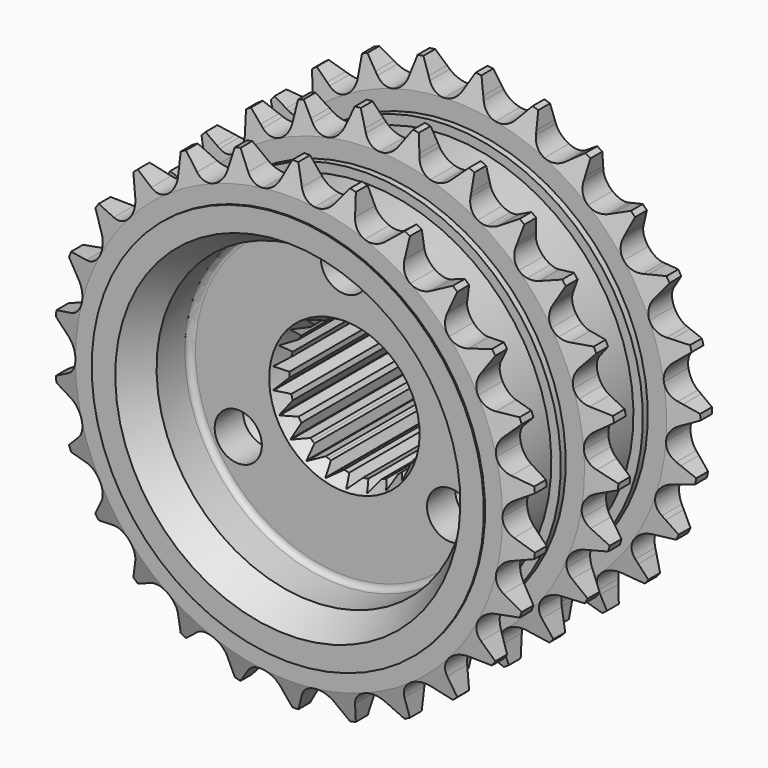
from build123d import *

# Parameters (mm, degrees)
F3_D      = 8
F3_DEPTH  = 6
F3_TIP    = 2.4034424761
F5_DEPTH  = 28.501
F6_R      = 41.9748747762
F7_DEPTH  = 6
F8_R      = 43.059736228
F9_DEPTH  = 6
F10_R     = 43.2062525831
F11_DEPTH = 6


# Not quite as in the source:
# - ends of sketch curves that miss each other by under 0.0002 mm in the source are joined


with BuildPart() as f1:
    # F0 (on Right) → F1 (revolve)
    with BuildSketch(Plane.YZ):
        with BuildLine():
            Line((0, 33.25), (0, 29.25))
            Line((0, 29.25), (5, 26.25))
            Line((5, 26.25), (11, 26.25))
            ThreePointArc((11, 26.25), (11.7071067812, 25.9571067812), (12, 25.25))
            Line((12, 25.25), (12, 12.75))
            Line((12, 12.75), (14.5, 11.35))
            Line((14.5, 11.35), (35.6, 11.35))
            Line((35.6, 11.35), (37, 12.75))
            Line((37, 12.75), (37, 17.5))
            Line((37, 17.5), (34.5, 18.75))
            ThreePointArc((34.5, 18.75), (31.5, 23.25), (34.5, 27.75))
            Line((34.5, 27.75), (37.5, 27.75))
            Line((37.5, 27.75), (40.5, 29.25))
            Line((40.5, 29.25), (40.5, 33.25))
            Line((40.5, 33.25), (40.25, 33.25))
            Line((40.25, 33.25), (40.25, 36.2))
            Line((40.25, 36.2), (38.9, 40.85))
            Line((38.9, 40.85), (36.4, 40.85))
            Line((36.4, 40.85), (35.05, 36.2))
            Line((35.05, 36.2), (35.05, 33))
            Line((35.05, 33), (34, 33))
            Line((34, 33), (34, 31.4))
            Line((34, 31.4), (23.9, 31.4))
            Line((23.9, 31.4), (23.9, 33))
            Line((23.9, 33), (22.85, 33))
            Line((22.85, 33), (22.85, 36.2))
            Line((22.85, 36.2), (21.5, 40.85))
            Line((21.5, 40.85), (19, 40.85))
            Line((19, 40.85), (17.65, 36.2))
            Line((17.65, 36.2), (17.65, 33))
            Line((17.65, 33), (16.6, 33))
            Line((16.6, 33), (16.6, 31.4))
            Line((16.6, 31.4), (6.5, 31.4))
            Line((6.5, 31.4), (6.5, 33))
            Line((6.5, 33), (5.45, 33))
            Line((5.45, 33), (5.45, 36.2))
            Line((5.45, 36.2), (4.1, 40.85))
            Line((4.1, 40.85), (1.6, 40.85))
            Line((1.6, 40.85), (0.25, 36.2))
            Line((0.25, 36.2), (0.25, 33.25))
            Line((0.25, 33.25), (0, 33.25))
        make_face()
    revolve(axis=Axis((0, 20.25, 0), (0, 1, 0)))

    # F3
    with Locations(Plane.XZ.offset(-12)):
        with Locations((0, 20.78), (17.9960078906, -10.39), (-17.9960078906, -10.39)):
            Hole(F3_D / 2, depth=F3_DEPTH)
            with Locations((0, 0, -(F3_DEPTH + F3_TIP / 2))):  # 118° drill point
                Cone(0, F3_D / 2, F3_TIP, mode=Mode.SUBTRACT)

    # F4 (on face) → F5 (cut, through all)
    with BuildSketch(Plane.XZ.offset(-12)):
        with BuildLine():
            Line((1.168584, 11.289682), (0.05, 12.4999))
            ThreePointArc((0.05, 12.4999), (0.02500005, 12.4999749999), (0, 12.5))
            ThreePointArc((0, 12.5), (-0.02500005, 12.4999749999), (-0.05, 12.4998999996))
            Line((-0.05, 12.4998999996), (-1.168584, 11.289682))
            ThreePointArc((-1.168584, 11.289682), (-1.3922022006, 11.2642919455), (-1.6152730599, 11.2344734163))
            ThreePointArc((-1.6152730599, 11.2344734163), (-1.8377093299, 11.2002376947), (-2.0594230559, 11.161598303))
            Line((-2.0594230559, 11.161598303), (-3.473654, 12.007653))
            ThreePointArc((-3.473654, 12.007653), (-3.497662502, 12.0006815232), (-3.5216570429, 11.993662146))
            ThreePointArc((-3.5216570429, 11.993662146), (-3.5456370746, 11.9865949183), (-3.5696029241, 11.9794797452))
            Line((-3.5696029241, 11.9794797452), (-4.301919, 10.503142))
            ThreePointArc((-4.301919, 10.503142), (-4.5093260475, 10.4157802683), (-4.7149601243, 10.3243232721))
            ThreePointArc((-4.7149601243, 10.3243232721), (-4.9187409108, 10.2288067658), (-5.1205877627, 10.1292685306))
            Line((-5.1205877627, 10.1292685306), (-6.715893, 10.542617))
            ThreePointArc((-6.715893, 10.542617), (-6.7369651285, 10.5291643), (-6.7580101367, 10.5156692127))
            ThreePointArc((-6.7580101367, 10.5156692127), (-6.7790281001, 10.5021320701), (-6.800018947, 10.4885529183))
            Line((-6.800018947, 10.4885529183), (-7.086738, 8.865701))
            ThreePointArc((-7.086738, 8.865701), (-7.2611308043, 8.7234442419), (-7.4326689778, 8.5777579744))
            ThreePointArc((-7.4326689778, 8.5777579744), (-7.6012851696, 8.4286988184), (-7.7669127104, 8.2763256914))
            Line((-7.7669127104, 8.2763256914), (-9.414051, 8.223481))
            ThreePointArc((-9.414051, 8.223481), (-9.4304793733, 8.2046364204), (-9.4468699032, 8.1857589161))
            ThreePointArc((-9.4468699032, 8.1857589161), (-9.4632224701, 8.1668488709), (-9.4795371845, 8.1479061585))
            Line((-9.4795371845, 8.1479061585), (-9.297432, 6.510013))
            ThreePointArc((-9.297432, 6.510013), (-9.4246825051, 6.3243861107), (-9.5482278417, 6.1362728983))
            ThreePointArc((-9.5482278417, 6.1362728983), (-9.668018783, 5.9457474561), (-9.7840084989, 5.7528842934))
            Line((-9.7840084989, 5.7528842934), (-11.349538, 5.238128))
            ThreePointArc((-11.349538, 5.238128), (-11.3599916731, 5.2154184096), (-11.3703998244, 5.1926879198))
            ThreePointArc((-11.3703998244, 5.1926879198), (-11.3807624714, 5.1699367084), (-11.3910795953, 5.1471648171))
            Line((-11.3910795953, 5.1471648171), (-10.754903, 3.626922))
            ThreePointArc((-10.754903, 3.626922), (-10.8247020133, 3.4129644481), (-10.8902451009, 3.1976650296))
            ThreePointArc((-10.8902451009, 3.1976650296), (-10.9515066301, 2.9811076013), (-11.0084622745, 2.7633780689))
            Line((-11.0084622745, 2.7633780689), (-12.365553, 1.828412))
            ThreePointArc((-12.365553, 1.828412), (-12.3691854533, 1.803677139), (-12.3727680904, 1.778935013))
            ThreePointArc((-12.3727680904, 1.778935013), (-12.3763012032, 1.7541860017), (-12.379784811, 1.7294299736))
            Line((-12.379784811, 1.7294299736), (-11.341076, 0.45))
            ThreePointArc((-11.341076, 0.45), (-11.3477687274, 0.2250442367), (-11.35, 0))
            ThreePointArc((-11.35, 0), (-11.3477687274, -0.2250442367), (-11.341075787, -0.4499999916))
            Line((-11.341075787, -0.4499999916), (-12.379785, -1.72943))
            ThreePointArc((-12.379785, -1.72943), (-12.3763012032, -1.7541860017), (-12.3727680904, -1.778935013))
            ThreePointArc((-12.3727680904, -1.778935013), (-12.3691854533, -1.803677139), (-12.3655533388, -1.8284120501))
            Line((-12.3655533388, -1.8284120501), (-11.008462, -2.763378))
            ThreePointArc((-11.008462, -2.763378), (-10.9515066301, -2.9811076013), (-10.8902451009, -3.1976650296))
            ThreePointArc((-10.8902451009, -3.1976650296), (-10.8247020133, -3.4129644481), (-10.7549029276, -3.6269219756))
            Line((-10.7549029276, -3.6269219756), (-11.39108, -5.147165))
            ThreePointArc((-11.39108, -5.147165), (-11.3807624714, -5.1699367084), (-11.3703998244, -5.1926879198))
            ThreePointArc((-11.3703998244, -5.1926879198), (-11.3599916731, -5.2154184096), (-11.3495380814, -5.2381280376))
            Line((-11.3495380814, -5.2381280376), (-9.784008, -5.752884))
            ThreePointArc((-9.784008, -5.752884), (-9.668018783, -5.9457474561), (-9.5482278417, -6.1362728983))
            ThreePointArc((-9.5482278417, -6.1362728983), (-9.4246825051, -6.3243861107), (-9.2974316011, -6.5100127207))
            Line((-9.2974316011, -6.5100127207), (-9.479537, -8.147906))
            ThreePointArc((-9.479537, -8.147906), (-9.4632224701, -8.1668488709), (-9.4468699032, -8.1857589161))
            ThreePointArc((-9.4468699032, -8.1857589161), (-9.4304793733, -8.2046364204), (-9.4140511209, -8.2234811056))
            Line((-9.4140511209, -8.2234811056), (-7.766913, -8.276326))
            ThreePointArc((-7.766913, -8.276326), (-7.6012851696, -8.4286988184), (-7.4326689778, -8.5777579744))
            ThreePointArc((-7.4326689778, -8.5777579744), (-7.2611308043, -8.7234442419), (-7.0867377331, -8.8657006661))
            Line((-7.0867377331, -8.8657006661), (-6.800019, -10.488553))
            ThreePointArc((-6.800019, -10.488553), (-6.7790281001, -10.5021320701), (-6.7580101367, -10.5156692127))
            ThreePointArc((-6.7580101367, -10.5156692127), (-6.7369651285, -10.5291643), (-6.715893172, -10.54261727))
            Line((-6.715893172, -10.54261727), (-5.120588, -10.129269))
            ThreePointArc((-5.120588, -10.129269), (-4.9187409108, -10.2288067658), (-4.7149601243, -10.3243232721))
            ThreePointArc((-4.7149601243, -10.3243232721), (-4.5093260475, -10.4157802683), (-4.3019190175, -10.5031420426))
            Line((-4.3019190175, -10.5031420426), (-3.569603, -11.97948))
            ThreePointArc((-3.569603, -11.97948), (-3.5456370746, -11.9865949183), (-3.5216570429, -11.993662146))
            ThreePointArc((-3.5216570429, -11.993662146), (-3.497662502, -12.0006815232), (-3.4736539702, -12.007652897))
            Line((-3.4736539702, -12.007652897), (-2.059423, -11.161598))
            ThreePointArc((-2.059423, -11.161598), (-1.8377093299, -11.2002376947), (-1.6152730599, -11.2344734163))
            ThreePointArc((-1.6152730599, -11.2344734163), (-1.3922022006, -11.2642919455), (-1.1685839627, -11.2896816395))
            Line((-1.1685839627, -11.2896816395), (-0.05, -12.4999))
            ThreePointArc((-0.05, -12.4999), (-0.02500005, -12.4999749999), (0, -12.5))
            ThreePointArc((0, -12.5), (0.02500005, -12.4999749999), (0.05, -12.4998999996))
            Line((0.05, -12.4998999996), (1.168584, -11.289682))
            ThreePointArc((1.168584, -11.289682), (1.3922022006, -11.2642919455), (1.6152730599, -11.2344734163))
            ThreePointArc((1.6152730599, -11.2344734163), (1.8377093299, -11.2002376947), (2.0594230559, -11.161598303))
            Line((2.0594230559, -11.161598303), (3.473654, -12.007653))
            ThreePointArc((3.473654, -12.007653), (3.497662502, -12.0006815232), (3.5216570429, -11.993662146))
            ThreePointArc((3.5216570429, -11.993662146), (3.5456370746, -11.9865949183), (3.5696029241, -11.9794797452))
            Line((3.5696029241, -11.9794797452), (4.301919, -10.503142))
            ThreePointArc((4.301919, -10.503142), (4.5093260475, -10.4157802683), (4.7149601243, -10.3243232721))
            ThreePointArc((4.7149601243, -10.3243232721), (4.9187409108, -10.2288067658), (5.1205877627, -10.1292685306))
            Line((5.1205877627, -10.1292685306), (6.715893, -10.542617))
            ThreePointArc((6.715893, -10.542617), (6.7369651285, -10.5291643), (6.7580101367, -10.5156692127))
            ThreePointArc((6.7580101367, -10.5156692127), (6.7790281001, -10.5021320701), (6.800018947, -10.4885529183))
            Line((6.800018947, -10.4885529183), (7.086738, -8.865701))
            ThreePointArc((7.086738, -8.865701), (7.2611308043, -8.7234442419), (7.4326689778, -8.5777579744))
            ThreePointArc((7.4326689778, -8.5777579744), (7.6012851696, -8.4286988184), (7.7669127104, -8.2763256914))
            Line((7.7669127104, -8.2763256914), (9.414051, -8.223481))
            ThreePointArc((9.414051, -8.223481), (9.4304793733, -8.2046364204), (9.4468699032, -8.1857589161))
            ThreePointArc((9.4468699032, -8.1857589161), (9.4632224701, -8.1668488709), (9.4795371845, -8.1479061585))
            Line((9.4795371845, -8.1479061585), (9.297432, -6.510013))
            ThreePointArc((9.297432, -6.510013), (9.4246825051, -6.3243861107), (9.5482278417, -6.1362728983))
            ThreePointArc((9.5482278417, -6.1362728983), (9.668018783, -5.9457474561), (9.7840084989, -5.7528842934))
            Line((9.7840084989, -5.7528842934), (11.349538, -5.238128))
            ThreePointArc((11.349538, -5.238128), (11.3599916731, -5.2154184096), (11.3703998244, -5.1926879198))
            ThreePointArc((11.3703998244, -5.1926879198), (11.3807624714, -5.1699367084), (11.3910795953, -5.1471648171))
            Line((11.3910795953, -5.1471648171), (10.754903, -3.626922))
            ThreePointArc((10.754903, -3.626922), (10.8247020133, -3.4129644481), (10.8902451009, -3.1976650296))
            ThreePointArc((10.8902451009, -3.1976650296), (10.9515066301, -2.9811076013), (11.0084622745, -2.7633780689))
            Line((11.0084622745, -2.7633780689), (12.365553, -1.828412))
            ThreePointArc((12.365553, -1.828412), (12.3691854533, -1.803677139), (12.3727680904, -1.778935013))
            ThreePointArc((12.3727680904, -1.778935013), (12.3763012032, -1.7541860017), (12.379784811, -1.7294299736))
            Line((12.379784811, -1.7294299736), (11.341076, -0.45))
            ThreePointArc((11.341076, -0.45), (11.3477687274, -0.2250442367), (11.35, 0))
            ThreePointArc((11.35, 0), (11.3477687274, 0.2250442367), (11.341075787, 0.4499999916))
            Line((11.341075787, 0.4499999916), (12.379785, 1.72943))
            ThreePointArc((12.379785, 1.72943), (12.3763012032, 1.7541860017), (12.3727680904, 1.778935013))
            ThreePointArc((12.3727680904, 1.778935013), (12.3691854533, 1.803677139), (12.3655533388, 1.8284120501))
            Line((12.3655533388, 1.8284120501), (11.008462, 2.763378))
            ThreePointArc((11.008462, 2.763378), (10.9515066301, 2.9811076013), (10.8902451009, 3.1976650296))
            ThreePointArc((10.8902451009, 3.1976650296), (10.8247020133, 3.4129644481), (10.7549029276, 3.6269219756))
            Line((10.7549029276, 3.6269219756), (11.39108, 5.147165))
            ThreePointArc((11.39108, 5.147165), (11.3807624714, 5.1699367084), (11.3703998244, 5.1926879198))
            ThreePointArc((11.3703998244, 5.1926879198), (11.3599916731, 5.2154184096), (11.3495380814, 5.2381280376))
            Line((11.3495380814, 5.2381280376), (9.784008, 5.752884))
            ThreePointArc((9.784008, 5.752884), (9.668018783, 5.9457474561), (9.5482278417, 6.1362728983))
            ThreePointArc((9.5482278417, 6.1362728983), (9.4246825051, 6.3243861107), (9.2974316011, 6.5100127207))
            Line((9.2974316011, 6.5100127207), (9.479537, 8.147906))
            ThreePointArc((9.479537, 8.147906), (9.4632224701, 8.1668488709), (9.4468699032, 8.1857589161))
            ThreePointArc((9.4468699032, 8.1857589161), (9.4304793733, 8.2046364204), (9.4140511209, 8.2234811056))
            Line((9.4140511209, 8.2234811056), (7.766913, 8.276326))
            ThreePointArc((7.766913, 8.276326), (7.6012851696, 8.4286988184), (7.4326689778, 8.5777579744))
            ThreePointArc((7.4326689778, 8.5777579744), (7.2611308043, 8.7234442419), (7.0867377331, 8.8657006661))
            Line((7.0867377331, 8.8657006661), (6.800019, 10.488553))
            ThreePointArc((6.800019, 10.488553), (6.7790281001, 10.5021320701), (6.7580101367, 10.5156692127))
            ThreePointArc((6.7580101367, 10.5156692127), (6.7369651285, 10.5291643), (6.715893172, 10.54261727))
            Line((6.715893172, 10.54261727), (5.120588, 10.129269))
            ThreePointArc((5.120588, 10.129269), (4.9187409108, 10.2288067658), (4.7149601243, 10.3243232721))
            ThreePointArc((4.7149601243, 10.3243232721), (4.5093260475, 10.4157802683), (4.3019190175, 10.5031420426))
            Line((4.3019190175, 10.5031420426), (3.569603, 11.97948))
            ThreePointArc((3.569603, 11.97948), (3.5456370746, 11.9865949183), (3.5216570429, 11.993662146))
            ThreePointArc((3.5216570429, 11.993662146), (3.497662502, 12.0006815232), (3.4736539702, 12.007652897))
            Line((3.4736539702, 12.007652897), (2.059423, 11.161598))
            ThreePointArc((2.059423, 11.161598), (1.8377093299, 11.2002376947), (1.6152730599, 11.2344734163))
            ThreePointArc((1.6152730599, 11.2344734163), (1.3922022006, 11.2642919455), (1.168584, 11.289682))
        make_face()
    extrude(amount=-F5_DEPTH, mode=Mode.SUBTRACT)

    # F6 (on face) → F7 (cut)
    with BuildSketch(Plane.XZ.offset(-0.25)):
        Circle(F6_R)
        with BuildLine():
            ThreePointArc((0, 40.85), (0.2500046815, 40.8492349703), (0.4999999989, 40.8469399099))
            Line((0.4999999989, 40.8469399099), (1.816578, 37.832086))
            ThreePointArc((1.816578, 37.832086), (2.8382605046, 36.5459186619), (4.3634280667, 35.936061549))
            ThreePointArc((4.3634280667, 35.936061549), (5.9902249889, 36.1632008832), (7.290019463, 37.1674897438))
            Line((7.290019463, 37.1674897438), (9.2898416715, 39.779659992))
            ThreePointArc((9.2898416715, 39.779659992), (9.5331218028, 39.722060479), (9.7760448861, 39.6629732419))
            ThreePointArc((9.7760448861, 39.6629732419), (10.0186018024, 39.6024004061), (10.2607834663, 39.5403442405))
            Line((10.2607834663, 39.5403442405), (10.8176023373, 36.2980187671))
            ThreePointArc((10.8176023373, 36.2980187671), (11.5017966143, 34.804720487), (12.8366972187, 33.8475882252))
            ThreePointArc((12.8366972187, 33.8475882252), (14.4705803796, 33.678809317), (15.9729472444, 34.3428541905))
            Line((15.9729472444, 34.3428541905), (18.5397915123, 36.4005307385))
            ThreePointArc((18.5397915123, 36.4005307385), (18.7622178993, 36.2863842164), (18.983941578, 36.1708786479))
            ThreePointArc((18.983941578, 36.1708786479), (19.2049542026, 36.0540182792), (19.425247495, 35.9358074872))
            Line((19.425247495, 35.9358074872), (19.1899469471, 32.6544426213))
            ThreePointArc((19.1899469471, 32.6544426213), (19.496890112, 31.0407984674), (20.563944188, 29.7920161047))
            ThreePointArc((20.563944188, 29.7920161047), (22.1099582371, 29.2371277708), (23.7275853913, 29.5223367829))
            Line((23.7275853913, 29.5223367829), (26.7122760597, 30.905934949))
            ThreePointArc((26.7122760597, 30.905934949), (26.9009220894, 30.7418751988), (27.0885605891, 30.5766640628))
            ThreePointArc((27.0885605891, 30.5766640628), (27.2751844718, 30.4103076609), (27.4607867473, 30.2428122241))
            Line((27.4607867473, 30.2428122241), (26.447041593, 27.1131089645))
            ThreePointArc((26.447041593, 27.1131089645), (26.3588952248, 25.4728980696), (27.0960894679, 24.0050402978))
            ThreePointArc((27.0960894679, 24.0050402978), (28.4643856883, 23.0962906312), (30.1032625215, 22.9860884708))
            Line((30.1032625215, 22.9860884708), (33.3323402178, 23.6151985588))
            ThreePointArc((33.3323402178, 23.6151985588), (33.4762424686, 23.4107601368), (33.6188909218, 23.205444904))
            ThreePointArc((33.6188909218, 23.205444904), (33.7602801607, 22.9992604983), (33.9004048897, 22.7922146426))
            Line((33.9004048897, 22.7922146426), (32.1671303126, 19.9960599668))
            ThreePointArc((32.1671303126, 19.9960599668), (31.6890171577, 18.4246054262), (32.0535085182, 16.8229788035))
            ThreePointArc((32.0535085182, 16.8229788035), (33.1645665071, 15.6131810318), (34.7294474548, 15.1139722478))
            Line((34.7294474548, 15.1139722478), (38.0152499205, 14.9520326661))
            ThreePointArc((38.0152499205, 14.9520326661), (38.1060453167, 14.7190967904), (38.1954135137, 14.4856096357))
            ThreePointArc((38.1954135137, 14.4856096357), (38.2833510803, 14.2515799145), (38.3698547229, 14.0170163925))
            Line((38.3698547229, 14.0170163925), (36.0177823412, 11.7169126465))
            ThreePointArc((36.0177823412, 11.7169126465), (35.1774885984, 10.3055416862), (35.1480941632, 8.6632269302))
            ThreePointArc((35.1480941632, 8.6632269302), (35.9373432688, 7.2226901023), (37.3372831385, 6.3634868948))
            Line((37.3372831385, 6.3634868948), (40.4888514776, 5.4199089832))
            ThreePointArc((40.4888514776, 5.4199089832), (40.5212633208, 5.1720130402), (40.5521575069, 4.9239233884))
            ThreePointArc((40.5521575069, 4.9239233884), (40.5815327895, 4.6756493084), (40.6093880683, 4.4272000994))
            Line((40.6093880683, 4.4272000994), (37.7752117794, 2.7568209525))
            ThreePointArc((37.7752117794, 2.7568209525), (36.6215722667, 1.5875573225), (36.2000003336, -2.027e-07))
            ThreePointArc((36.2000003336, -2.027e-07), (36.6215722667, -1.5875573225), (37.7752116417, -2.7568211861))
            Line((37.7752116417, -2.7568211861), (40.6093881579, -4.4272001091))
            ThreePointArc((40.6093881579, -4.4272001091), (40.5815327895, -4.6756493084), (40.5521575069, -4.9239233884))
            ThreePointArc((40.5521575069, -4.9239233884), (40.5212633208, -5.1720130402), (40.4888513883, -5.4199089713))
            Line((40.4888513883, -5.4199089713), (37.3372832163, -6.3634871547))
            ThreePointArc((37.3372832163, -6.3634871547), (35.9373432688, -7.2226901023), (35.1480940662, -8.6632273238))
            ThreePointArc((35.1480940662, -8.6632273238), (35.1774885984, -10.3055416862), (36.0177821515, -11.7169128404))
            Line((36.0177821515, -11.7169128404), (38.3698548075, -14.0170164234))
            ThreePointArc((38.3698548075, -14.0170164234), (38.2833510803, -14.2515799145), (38.1954135137, -14.4856096357))
            ThreePointArc((38.1954135137, -14.4856096357), (38.1060453167, -14.7190967904), (38.0152498366, -14.9520326331))
            Line((38.0152498366, -14.9520326331), (34.7294474682, -15.1139725187))
            ThreePointArc((34.7294474682, -15.1139725187), (33.1645665071, -15.6131810318), (32.0535083298, -16.8229791625))
            ThreePointArc((32.0535083298, -16.8229791625), (31.6890171577, -18.4246054262), (32.1671300821, -19.9960601097))
            Line((32.1671300821, -19.9960601097), (33.9004049645, -22.7922146929))
            ThreePointArc((33.9004049645, -22.7922146929), (33.7602801607, -22.9992604983), (33.6188909218, -23.205444904))
            ThreePointArc((33.6188909218, -23.205444904), (33.4762424686, -23.4107601368), (33.3323401442, -23.6151985067))
            Line((33.3323401442, -23.6151985067), (30.1032624696, -22.986088737))
            ThreePointArc((30.1032624696, -22.986088737), (28.4643856883, -23.0962906312), (27.096089199, -24.0050406012))
            ThreePointArc((27.096089199, -24.0050406012), (26.3588952248, -25.4728980696), (26.447041335, -27.113109048))
            Line((26.447041335, -27.113109048), (27.4607868079, -30.2428122908))
            ThreePointArc((27.4607868079, -30.2428122908), (27.2751844718, -30.4103076609), (27.0885605891, -30.5766640628))
            ThreePointArc((27.0885605891, -30.5766640628), (26.9009220894, -30.7418751988), (26.7122760008, -30.9059348808))
            Line((26.7122760008, -30.9059348808), (23.7275852772, -29.522337029))
            ThreePointArc((23.7275852772, -29.522337029), (22.1099582371, -29.2371277708), (20.5639438543, -29.792016335))
            ThreePointArc((20.5639438543, -29.792016335), (19.496890112, -31.0407984674), (19.1899466766, -32.6544426407))
            Line((19.1899466766, -32.6544426407), (19.4252475379, -35.9358075665))
            ThreePointArc((19.4252475379, -35.9358075665), (19.2049542026, -36.0540182792), (18.983941578, -36.1708786479))
            ThreePointArc((18.983941578, -36.1708786479), (18.7622178993, -36.2863842164), (18.5397914713, -36.4005306582))
            Line((18.5397914713, -36.4005306582), (15.9729470748, -34.3428544022))
            ThreePointArc((15.9729470748, -34.3428544022), (14.4705803796, -33.678809317), (12.8366968397, -33.847588369))
            ThreePointArc((12.8366968397, -33.847588369), (11.5017966143, -34.804720487), (10.81760207, -36.2980187212))
            Line((10.81760207, -36.2980187212), (10.2607834889, -39.5403443277))
            ThreePointArc((10.2607834889, -39.5403443277), (10.0186018024, -39.6024004061), (9.7760448861, -39.6629732419))
            ThreePointArc((9.7760448861, -39.6629732419), (9.5331218028, -39.722060479), (9.289841651, -39.7796599043))
            Line((9.289841651, -39.7796599043), (7.2900192477, -37.1674899087))
            ThreePointArc((7.2900192477, -37.1674899087), (5.9902249889, -36.1632008832), (4.3634276642, -35.9360615979))
            ThreePointArc((4.3634276642, -35.9360615979), (2.8382605046, -36.5459186619), (1.8165777515, -37.8320858915))
            Line((1.8165777515, -37.8320858915), (0.5, -40.84694))
            ThreePointArc((0.5, -40.84694), (0.2500046815, -40.8492349703), (0, -40.85))
            ThreePointArc((0, -40.85), (-0.2500046815, -40.8492349703), (-0.4999999989, -40.8469399099))
            Line((-0.4999999989, -40.8469399099), (-1.816578, -37.832086))
            ThreePointArc((-1.816578, -37.832086), (-2.8382605046, -36.5459186619), (-4.3634280667, -35.936061549))
            ThreePointArc((-4.3634280667, -35.936061549), (-5.9902249889, -36.1632008832), (-7.290019463, -37.1674897438))
            Line((-7.290019463, -37.1674897438), (-9.2898416715, -39.779659992))
            ThreePointArc((-9.2898416715, -39.779659992), (-9.5331218028, -39.722060479), (-9.7760448861, -39.6629732419))
            ThreePointArc((-9.7760448861, -39.6629732419), (-10.0186018024, -39.6024004061), (-10.2607834663, -39.5403442405))
            Line((-10.2607834663, -39.5403442405), (-10.8176023373, -36.2980187671))
            ThreePointArc((-10.8176023373, -36.2980187671), (-11.5017966143, -34.804720487), (-12.8366972187, -33.8475882252))
            ThreePointArc((-12.8366972187, -33.8475882252), (-14.4705803796, -33.678809317), (-15.9729472444, -34.3428541905))
            Line((-15.9729472444, -34.3428541905), (-18.5397915123, -36.4005307385))
            ThreePointArc((-18.5397915123, -36.4005307385), (-18.7622178993, -36.2863842164), (-18.983941578, -36.1708786479))
            ThreePointArc((-18.983941578, -36.1708786479), (-19.2049542026, -36.0540182792), (-19.425247495, -35.9358074872))
            Line((-19.425247495, -35.9358074872), (-19.1899469471, -32.6544426213))
            ThreePointArc((-19.1899469471, -32.6544426213), (-19.496890112, -31.0407984674), (-20.563944188, -29.7920161047))
            ThreePointArc((-20.563944188, -29.7920161047), (-22.1099582371, -29.2371277708), (-23.7275853913, -29.5223367829))
            Line((-23.7275853913, -29.5223367829), (-26.7122760597, -30.905934949))
            ThreePointArc((-26.7122760597, -30.905934949), (-26.9009220894, -30.7418751988), (-27.0885605891, -30.5766640628))
            ThreePointArc((-27.0885605891, -30.5766640628), (-27.2751844718, -30.4103076609), (-27.4607867473, -30.2428122241))
            Line((-27.4607867473, -30.2428122241), (-26.447041593, -27.1131089645))
            ThreePointArc((-26.447041593, -27.1131089645), (-26.3588952248, -25.4728980696), (-27.0960894679, -24.0050402978))
            ThreePointArc((-27.0960894679, -24.0050402978), (-28.4643856883, -23.0962906312), (-30.1032625215, -22.9860884708))
            Line((-30.1032625215, -22.9860884708), (-33.3323402178, -23.6151985588))
            ThreePointArc((-33.3323402178, -23.6151985588), (-33.4762424686, -23.4107601368), (-33.6188909218, -23.205444904))
            ThreePointArc((-33.6188909218, -23.205444904), (-33.7602801607, -22.9992604983), (-33.9004048897, -22.7922146426))
            Line((-33.9004048897, -22.7922146426), (-32.1671303126, -19.9960599668))
            ThreePointArc((-32.1671303126, -19.9960599668), (-31.6890171577, -18.4246054262), (-32.0535085182, -16.8229788035))
            ThreePointArc((-32.0535085182, -16.8229788035), (-33.1645665071, -15.6131810318), (-34.7294474548, -15.1139722478))
            Line((-34.7294474548, -15.1139722478), (-38.0152499205, -14.9520326661))
            ThreePointArc((-38.0152499205, -14.9520326661), (-38.1060453167, -14.7190967904), (-38.1954135137, -14.4856096357))
            ThreePointArc((-38.1954135137, -14.4856096357), (-38.2833510803, -14.2515799145), (-38.3698547229, -14.0170163925))
            Line((-38.3698547229, -14.0170163925), (-36.0177823412, -11.7169126465))
            ThreePointArc((-36.0177823412, -11.7169126465), (-35.1774885984, -10.3055416862), (-35.1480941632, -8.6632269302))
            ThreePointArc((-35.1480941632, -8.6632269302), (-35.9373432688, -7.2226901023), (-37.3372831385, -6.3634868948))
            Line((-37.3372831385, -6.3634868948), (-40.4888514776, -5.4199089832))
            ThreePointArc((-40.4888514776, -5.4199089832), (-40.5212633208, -5.1720130402), (-40.5521575069, -4.9239233884))
            ThreePointArc((-40.5521575069, -4.9239233884), (-40.5815327895, -4.6756493084), (-40.6093880683, -4.4272000994))
            Line((-40.6093880683, -4.4272000994), (-37.7752117794, -2.7568209525))
            ThreePointArc((-37.7752117794, -2.7568209525), (-36.6215722667, -1.5875573225), (-36.2000003336, 2.027e-07))
            ThreePointArc((-36.2000003336, 2.027e-07), (-36.6215722667, 1.5875573225), (-37.7752116417, 2.7568211861))
            Line((-37.7752116417, 2.7568211861), (-40.6093881579, 4.4272001091))
            ThreePointArc((-40.6093881579, 4.4272001091), (-40.5815327895, 4.6756493084), (-40.5521575069, 4.9239233884))
            ThreePointArc((-40.5521575069, 4.9239233884), (-40.5212633208, 5.1720130402), (-40.4888513883, 5.4199089713))
            Line((-40.4888513883, 5.4199089713), (-37.3372832163, 6.3634871547))
            ThreePointArc((-37.3372832163, 6.3634871547), (-35.9373432688, 7.2226901023), (-35.1480940662, 8.6632273238))
            ThreePointArc((-35.1480940662, 8.6632273238), (-35.1774885984, 10.3055416862), (-36.0177821515, 11.7169128404))
            Line((-36.0177821515, 11.7169128404), (-38.3698548075, 14.0170164234))
            ThreePointArc((-38.3698548075, 14.0170164234), (-38.2833510803, 14.2515799145), (-38.1954135137, 14.4856096357))
            ThreePointArc((-38.1954135137, 14.4856096357), (-38.1060453167, 14.7190967904), (-38.0152498366, 14.9520326331))
            Line((-38.0152498366, 14.9520326331), (-34.7294474682, 15.1139725187))
            ThreePointArc((-34.7294474682, 15.1139725187), (-33.1645665071, 15.6131810318), (-32.0535083298, 16.8229791625))
            ThreePointArc((-32.0535083298, 16.8229791625), (-31.6890171577, 18.4246054262), (-32.1671300821, 19.9960601097))
            Line((-32.1671300821, 19.9960601097), (-33.9004049645, 22.7922146929))
            ThreePointArc((-33.9004049645, 22.7922146929), (-33.7602801607, 22.9992604983), (-33.6188909218, 23.205444904))
            ThreePointArc((-33.6188909218, 23.205444904), (-33.4762424686, 23.4107601368), (-33.3323401442, 23.6151985067))
            Line((-33.3323401442, 23.6151985067), (-30.1032624696, 22.986088737))
            ThreePointArc((-30.1032624696, 22.986088737), (-28.4643856883, 23.0962906312), (-27.096089199, 24.0050406012))
            ThreePointArc((-27.096089199, 24.0050406012), (-26.3588952248, 25.4728980696), (-26.447041335, 27.113109048))
            Line((-26.447041335, 27.113109048), (-27.4607868079, 30.2428122908))
            ThreePointArc((-27.4607868079, 30.2428122908), (-27.2751844718, 30.4103076609), (-27.0885605891, 30.5766640628))
            ThreePointArc((-27.0885605891, 30.5766640628), (-26.9009220894, 30.7418751988), (-26.7122760008, 30.9059348808))
            Line((-26.7122760008, 30.9059348808), (-23.7275852772, 29.522337029))
            ThreePointArc((-23.7275852772, 29.522337029), (-22.1099582371, 29.2371277708), (-20.5639438543, 29.792016335))
            ThreePointArc((-20.5639438543, 29.792016335), (-19.496890112, 31.0407984674), (-19.1899466766, 32.6544426407))
            Line((-19.1899466766, 32.6544426407), (-19.4252475379, 35.9358075665))
            ThreePointArc((-19.4252475379, 35.9358075665), (-19.2049542026, 36.0540182792), (-18.983941578, 36.1708786479))
            ThreePointArc((-18.983941578, 36.1708786479), (-18.7622178993, 36.2863842164), (-18.5397914713, 36.4005306582))
            Line((-18.5397914713, 36.4005306582), (-15.9729470748, 34.3428544022))
            ThreePointArc((-15.9729470748, 34.3428544022), (-14.4705803796, 33.678809317), (-12.8366968397, 33.847588369))
            ThreePointArc((-12.8366968397, 33.847588369), (-11.5017966143, 34.804720487), (-10.81760207, 36.2980187212))
            Line((-10.81760207, 36.2980187212), (-10.2607834889, 39.5403443277))
            ThreePointArc((-10.2607834889, 39.5403443277), (-10.0186018024, 39.6024004061), (-9.7760448861, 39.6629732419))
            ThreePointArc((-9.7760448861, 39.6629732419), (-9.5331218028, 39.722060479), (-9.289841651, 39.7796599043))
            Line((-9.289841651, 39.7796599043), (-7.2900192477, 37.1674899087))
            ThreePointArc((-7.2900192477, 37.1674899087), (-5.9902249889, 36.1632008832), (-4.3634276642, 35.9360615979))
            ThreePointArc((-4.3634276642, 35.9360615979), (-2.8382605046, 36.5459186619), (-1.8165777515, 37.8320858915))
            Line((-1.8165777515, 37.8320858915), (-0.5, 40.84694))
            ThreePointArc((-0.5, 40.84694), (-0.2500046815, 40.8492349703), (0, 40.85))
        make_face(mode=Mode.SUBTRACT)
    extrude(amount=-F7_DEPTH, mode=Mode.SUBTRACT)

    # F8 (on face) → F9 (cut)
    with BuildSketch(Plane.XZ.offset(-17.65)):
        Circle(F8_R)
        with BuildLine():
            ThreePointArc((-1.266972328, 37.8544780474), (-0.1440496259, 36.6556839527), (1.4256736099, 36.1719157853))
            ThreePointArc((1.4256736099, 36.1719157853), (2.1960466062, 36.2349767214), (2.9288257676, 36.4809174875))
            ThreePointArc((2.9288257676, 36.4809174875), (3.6662000409, 36.9675825991), (4.2423923941, 37.63733339))
            Line((4.2423923941, 37.63733339), (6.023094, 40.403525))
            ThreePointArc((6.023094, 40.403525), (6.2702534613, 40.365906673), (6.5171780554, 40.3267763427))
            ThreePointArc((6.5171780554, 40.3267763427), (6.76385868, 40.2861355277), (7.0102859602, 40.2439857713))
            Line((7.0102859602, 40.2439857713), (7.672447, 37.667017))
            Line((7.672447, 37.667017), (7.829013, 37.057702))
            ThreePointArc((7.829013, 37.057702), (8.6324155495, 35.6250097279), (10.0407521805, 34.7796396253))
            ThreePointArc((10.0407521805, 34.7796396253), (10.8038310075, 34.6565057999), (11.574174416, 34.7199344425))
            ThreePointArc((11.574174416, 34.7199344425), (12.4065885176, 35.0159927365), (13.1263196236, 35.5283899308))
            Line((13.1263196236, 35.5283899308), (15.5172702598, 37.7880512522))
            ThreePointArc((15.5172702598, 37.7880512522), (15.7482450614, 37.6923769148), (15.9786299746, 37.5952907175))
            ThreePointArc((15.9786299746, 37.5952907175), (16.2084165249, 37.4967963132), (16.4375959793, 37.3968974438))
            Line((16.4375959793, 37.3968974438), (16.4638068294, 34.7363451925))
            Line((16.4638068294, 34.7363451925), (16.470004682, 34.1072670827))
            ThreePointArc((16.470004682, 34.1072670827), (16.9071961107, 32.5239394294), (18.0722987311, 31.3660972292))
            ThreePointArc((18.0722987311, 31.3660972292), (18.783736021, 31.0639247326), (19.5468741178, 30.9411550096))
            ThreePointArc((19.5468741178, 30.9411550096), (20.4259511657, 31.0294006539), (21.2473928688, 31.3546655893))
            Line((21.2473928688, 31.3546655893), (24.1096391751, 32.9764733197))
            ThreePointArc((24.1096391751, 32.9764733197), (24.3110059011, 32.8283032165), (24.5114619997, 32.6789034491))
            ThreePointArc((24.5114619997, 32.6789034491), (24.7110001167, 32.5282795923), (24.9096126683, 32.3764373691))
            Line((24.9096126683, 32.3764373691), (24.2983500493, 29.7869232639))
            Line((24.2983500493, 29.7869232639), (24.1538195579, 29.1746417774))
            ThreePointArc((24.1538195579, 29.1746417774), (24.1993918891, 27.5326959909), (25.0535489696, 26.1296712733))
            ThreePointArc((25.0535489696, 26.1296712733), (25.671998573, 25.6660212726), (26.3835805459, 25.364188114))
            ThreePointArc((26.3835805459, 25.364188114), (27.2582317774, 25.2394925926), (28.1336448716, 25.3587220532))
            Line((28.1336448716, 25.3587220532), (31.3008434965, 26.2484226224))
            ThreePointArc((31.3008434965, 26.2484226224), (31.4608994448, 26.0563678613), (31.6197769489, 25.8633370953))
            ThreePointArc((31.6197769489, 25.8633370953), (31.7774702025, 25.6693374969), (31.9339732118, 25.4743764381))
            Line((31.9339732118, 25.4743764381), (30.7207614853, 23.1063936262))
            Line((30.7207614853, 23.1063936262), (30.4339022366, 22.5464923376))
            ThreePointArc((30.4339022366, 22.5464923376), (30.0852069721, 20.9413523388), (30.5787780079, 19.3746838004))
            ThreePointArc((30.5787780079, 19.3746838004), (31.0682978819, 18.7765019484), (31.6869691731, 18.3131468003))
            ThreePointArc((31.6869691731, 18.3131468003), (32.5063630379, 17.9827569637), (33.3848716962, 17.8890217667))
            Line((33.3848716962, 17.8890217667), (36.6729565679, 17.9949090114))
            ThreePointArc((36.6729565679, 17.9949090114), (36.7823998684, 17.7701311171), (36.890465395, 17.5446875989))
            ThreePointArc((36.890465395, 17.5446875989), (36.9971492265, 17.3185868105), (37.1024473075, 17.0918373441))
            Line((37.1024473075, 17.0918373441), (35.3577939292, 15.0830043793))
            Line((35.3577939292, 15.0830043793), (34.9452771401, 14.6080227162))
            ThreePointArc((34.9452771401, 14.6080227162), (34.2225791812, 13.1329734074), (34.3268796177, 11.4937101292))
            ThreePointArc((34.3268796177, 11.4937101292), (34.6590206466, 10.7957605808), (35.1488263294, 10.1978119602))
            ThreePointArc((35.1488263294, 10.1978119602), (35.8653426344, 9.6809288646), (36.6958911267, 9.379676559))
            Line((36.6958911267, 9.379676559), (39.9137707043, 8.6955966975))
            ThreePointArc((39.9137707043, 8.6955966975), (39.9662409103, 8.4511589441), (40.0172140837, 8.2064046315))
            ThreePointArc((40.0172140837, 8.2064046315), (40.0666884166, 7.9613428092), (40.1146620276, 7.7159827899))
            Line((40.1146620276, 7.7159827899), (37.9399599103, 6.1830457424))
            Line((37.9399599103, 6.1830457424), (37.4257595571, 5.8205879126))
            ThreePointArc((37.4257595571, 5.8205879126), (36.3710594822, 4.561353798), (36.0800277572, 2.9447638031))
            ThreePointArc((36.0800277572, 2.9447638031), (36.2354871117, 2.1876088492), (36.5679614601, 1.4898173564))
            ThreePointArc((36.5679614601, 1.4898173564), (37.1399588822, 0.8164803688), (37.8742787492, 0.3252186435))
            Line((37.8742787492, 0.3252186435), (40.834941568, -1.1090720892))
            ThreePointArc((40.834941568, -1.1090720892), (40.8273893019, -1.358963868), (40.8183077466, -1.6088047439))
            ThreePointArc((40.8183077466, -1.6088047439), (40.8076973125, -1.8585854979), (40.7955584015, -2.1082966375))
            Line((40.7955584015, -2.1082966375), (38.3171933275, -3.0762490386))
            Line((38.3171933275, -3.0762490386), (37.7311928658, -3.3051183036))
            ThreePointArc((37.7311928658, -3.3051183036), (36.4057860096, -4.2753551142), (35.7363358291, -5.7753214913))
            ThreePointArc((35.7363358291, -5.7753214913), (35.7060787765, -6.5476787571), (35.86189959, -7.3047600168))
            ThreePointArc((35.86189959, -7.3047600168), (36.256135718, -8.0954189984), (36.8515509581, -8.7481397975))
            Line((36.8515509581, -8.7481397975), (39.3829340567, -10.8492856374))
            ThreePointArc((39.3829340567, -10.8492856374), (39.3157982287, -11.0901086397), (39.2471897317, -11.3305162354))
            ThreePointArc((39.2471897317, -11.3305162354), (39.1771111705, -11.5704995716), (39.1055652069, -11.8100495277))
            Line((39.1055652069, -11.8100495277), (36.4675707459, -12.1567634072))
            Line((36.4675707459, -12.1567634072), (35.8438263924, -12.2387430575))
            ThreePointArc((35.8438263924, -12.2387430575), (34.3247405838, -12.8635959276), (33.3157779589, -14.1597660931))
            ThreePointArc((33.3157779589, -14.1597660931), (33.1015629291, -14.9024390738), (33.0716744684, -15.6748112895))
            ThreePointArc((33.0716744684, -15.6748112895), (33.2652377316, -16.536842039), (33.6871449753, -17.3130881517))
            Line((33.6871449753, -17.3130881517), (35.6421335692, -19.95897814))
            ThreePointArc((35.6421335692, -19.95897814), (35.5193158696, -20.1767366082), (35.3951677074, -20.3937393081))
            ThreePointArc((35.3951677074, -20.3937393081), (35.2696937303, -20.6099782672), (35.1428987055, -20.8254452672))
            Line((35.1428987055, -20.8254452672), (32.4985855067, -20.5307708747))
            Line((32.4985855067, -20.5307708747), (31.8733470161, -20.461096551))
            ThreePointArc((31.8733470161, -20.461096551), (30.2488660006, -20.7042513029), (28.9590281716, -21.7212965583))
            ThreePointArc((28.9590281716, -21.7212965583), (28.5733045636, -22.3911237997), (28.3594438373, -23.1338995058))
            ThreePointArc((28.3594438373, -23.1338995058), (28.3410850425, -24.0172039292), (28.5649645744, -24.871862753))
            Line((28.5649645744, -24.871862753), (29.8299418326, -27.9087273809))
            ThreePointArc((29.8299418326, -27.9087273809), (29.6585799796, -28.0907659844), (29.4861071921, -28.2717523803))
            ThreePointArc((29.4861071921, -28.2717523803), (29.3125298906, -28.4516799401), (29.1378546705, -28.6305418251))
            Line((29.1378546705, -28.6305418251), (26.6409006055, -27.7116045651))
            Line((26.6409006055, -27.7116045651), (26.0505045661, -27.4943254859))
            ThreePointArc((26.0505045661, -27.4943254859), (24.4150372755, -27.3416508493), (22.9192849288, -28.0204642212))
            ThreePointArc((22.9192849288, -28.0204642212), (22.3844695966, -28.5785177989), (21.9990654128, -29.2485295711))
            ThreePointArc((21.9990654128, -29.2485295711), (21.7698515063, -30.1017732261), (21.7826922617, -30.9851750966))
            Line((21.7826922617, -30.9851750966), (22.2841423041, -34.2365228306))
            ThreePointArc((22.2841423041, -34.2365228306), (22.0741952258, -34.3722621475), (21.8634213045, -34.5067139679))
            ThreePointArc((21.8634213045, -34.5067139679), (21.6518283603, -34.6398733926), (21.4394244339, -34.77173536))
            Line((21.4394244339, -34.77173536), (19.2349433968, -33.2819405259))
            Line((19.2349433968, -33.2819405259), (18.7137014805, -32.9296841615))
            ThreePointArc((18.7137014805, -32.9296841615), (17.1622953291, -32.3900530313), (15.5475561542, -32.6911843538))
            ThreePointArc((15.5475561542, -32.6911843538), (14.8947306208, -33.1050322222), (14.3601812699, -33.6633414117))
            ThreePointArc((14.3601812699, -33.6633414117), (13.9334333308, -34.4369368786), (13.7344890517, -35.2977416902))
            Line((13.7344890517, -35.2977416902), (13.4432694244, -38.5746160181))
            ThreePointArc((13.4432694244, -38.5746160181), (13.2069384818, -38.6561673726), (12.9701128409, -38.7362707665))
            ThreePointArc((12.9701128409, -38.7362707665), (12.732801267, -38.8149233143), (12.4950127783, -38.8921220258))
            Line((12.4950127783, -38.8921220258), (10.711121194, -36.9180510782))
            Line((10.711121194, -36.9180510782), (10.2893260863, -36.4512892881))
            ThreePointArc((10.2893260863, -36.4512892881), (8.9121431606, -35.5560630641), (7.2722599289, -35.4620116793))
            ThreePointArc((7.2722599289, -35.4620116793), (6.5393640415, -35.7076025047), (5.8867355886, -36.1217622108))
            ThreePointArc((5.8867355886, -36.1217622108), (5.2872546561, -36.7707509329), (4.8880872609, -37.5589318388))
            Line((4.8880872609, -37.5589318388), (3.82112259, -40.6708927356))
            ThreePointArc((3.82112259, -40.6708927356), (3.5721424786, -40.6935166594), (3.3230285634, -40.7146163087))
            ThreePointArc((3.3230285634, -40.7146163087), (3.0737900459, -40.7341909795), (2.8244363976, -40.7522399266))
            Line((2.8244363976, -40.7522399266), (1.5648075608, -38.4086186935))
            Line((1.5648075608, -38.4086186935), (1.2669724602, -37.8544779763))
            ThreePointArc((1.2669724602, -37.8544779763), (0.1440496259, -36.6556839527), (-1.4256736099, -36.1719157853))
            ThreePointArc((-1.4256736099, -36.1719157853), (-2.1960466062, -36.2349767214), (-2.9288257676, -36.4809174875))
            ThreePointArc((-2.9288257676, -36.4809174875), (-3.6662000409, -36.9675825991), (-4.2423923941, -37.63733339))
            Line((-4.2423923941, -37.63733339), (-6.023094, -40.403525))
            ThreePointArc((-6.023094, -40.403525), (-6.2702534613, -40.365906673), (-6.5171780554, -40.3267763427))
            ThreePointArc((-6.5171780554, -40.3267763427), (-6.76385868, -40.2861355277), (-7.0102859602, -40.2439857713))
            Line((-7.0102859602, -40.2439857713), (-7.672447, -37.667017))
            Line((-7.672447, -37.667017), (-7.829013, -37.057702))
            ThreePointArc((-7.829013, -37.057702), (-8.6324155495, -35.6250097279), (-10.0407521805, -34.7796396253))
            ThreePointArc((-10.0407521805, -34.7796396253), (-10.8038310075, -34.6565057999), (-11.574174416, -34.7199344425))
            ThreePointArc((-11.574174416, -34.7199344425), (-12.4065885176, -35.0159927365), (-13.1263196236, -35.5283899308))
            Line((-13.1263196236, -35.5283899308), (-15.5172702598, -37.7880512522))
            ThreePointArc((-15.5172702598, -37.7880512522), (-15.7482450614, -37.6923769148), (-15.9786299746, -37.5952907175))
            ThreePointArc((-15.9786299746, -37.5952907175), (-16.2084165249, -37.4967963132), (-16.4375959793, -37.3968974438))
            Line((-16.4375959793, -37.3968974438), (-16.4638068294, -34.7363451925))
            Line((-16.4638068294, -34.7363451925), (-16.470004682, -34.1072670827))
            ThreePointArc((-16.470004682, -34.1072670827), (-16.9071961107, -32.5239394294), (-18.0722987311, -31.3660972292))
            ThreePointArc((-18.0722987311, -31.3660972292), (-18.783736021, -31.0639247326), (-19.5468741178, -30.9411550096))
            ThreePointArc((-19.5468741178, -30.9411550096), (-20.4259511657, -31.0294006539), (-21.2473928688, -31.3546655893))
            Line((-21.2473928688, -31.3546655893), (-24.1096391751, -32.9764733197))
            ThreePointArc((-24.1096391751, -32.9764733197), (-24.3110059011, -32.8283032165), (-24.5114619997, -32.6789034491))
            ThreePointArc((-24.5114619997, -32.6789034491), (-24.7110001167, -32.5282795923), (-24.9096126683, -32.3764373691))
            Line((-24.9096126683, -32.3764373691), (-24.2983500493, -29.7869232639))
            Line((-24.2983500493, -29.7869232639), (-24.1538195579, -29.1746417774))
            ThreePointArc((-24.1538195579, -29.1746417774), (-24.1993918891, -27.5326959909), (-25.0535489696, -26.1296712733))
            ThreePointArc((-25.0535489696, -26.1296712733), (-25.671998573, -25.6660212726), (-26.3835805459, -25.364188114))
            ThreePointArc((-26.3835805459, -25.364188114), (-27.2582317774, -25.2394925926), (-28.1336448716, -25.3587220532))
            Line((-28.1336448716, -25.3587220532), (-31.3008434965, -26.2484226224))
            ThreePointArc((-31.3008434965, -26.2484226224), (-31.4608994448, -26.0563678613), (-31.6197769489, -25.8633370953))
            ThreePointArc((-31.6197769489, -25.8633370953), (-31.7774702025, -25.6693374969), (-31.9339732118, -25.4743764381))
            Line((-31.9339732118, -25.4743764381), (-30.7207614853, -23.1063936262))
            Line((-30.7207614853, -23.1063936262), (-30.4339022366, -22.5464923376))
            ThreePointArc((-30.4339022366, -22.5464923376), (-30.0852069721, -20.9413523388), (-30.5787780079, -19.3746838004))
            ThreePointArc((-30.5787780079, -19.3746838004), (-31.0682978819, -18.7765019484), (-31.6869691731, -18.3131468003))
            ThreePointArc((-31.6869691731, -18.3131468003), (-32.5063630379, -17.9827569637), (-33.3848716962, -17.8890217667))
            Line((-33.3848716962, -17.8890217667), (-36.6729565679, -17.9949090114))
            ThreePointArc((-36.6729565679, -17.9949090114), (-36.7823998684, -17.7701311171), (-36.890465395, -17.5446875989))
            ThreePointArc((-36.890465395, -17.5446875989), (-36.9971492265, -17.3185868105), (-37.1024473075, -17.0918373441))
            Line((-37.1024473075, -17.0918373441), (-35.3577939292, -15.0830043793))
            Line((-35.3577939292, -15.0830043793), (-34.9452771401, -14.6080227162))
            ThreePointArc((-34.9452771401, -14.6080227162), (-34.2225791812, -13.1329734074), (-34.3268796177, -11.4937101292))
            ThreePointArc((-34.3268796177, -11.4937101292), (-34.6590206466, -10.7957605808), (-35.1488263294, -10.1978119602))
            ThreePointArc((-35.1488263294, -10.1978119602), (-35.8653426344, -9.6809288646), (-36.6958911267, -9.379676559))
            Line((-36.6958911267, -9.379676559), (-39.9137707043, -8.6955966975))
            ThreePointArc((-39.9137707043, -8.6955966975), (-39.9662409103, -8.4511589441), (-40.0172140837, -8.2064046315))
            ThreePointArc((-40.0172140837, -8.2064046315), (-40.0666884166, -7.9613428092), (-40.1146620276, -7.7159827899))
            Line((-40.1146620276, -7.7159827899), (-37.9399599103, -6.1830457424))
            Line((-37.9399599103, -6.1830457424), (-37.4257595571, -5.8205879126))
            ThreePointArc((-37.4257595571, -5.8205879126), (-36.3710594822, -4.561353798), (-36.0800277572, -2.9447638031))
            ThreePointArc((-36.0800277572, -2.9447638031), (-36.2354871117, -2.1876088492), (-36.5679614601, -1.4898173564))
            ThreePointArc((-36.5679614601, -1.4898173564), (-37.1399588822, -0.8164803688), (-37.8742787492, -0.3252186435))
            Line((-37.8742787492, -0.3252186435), (-40.834941568, 1.1090720892))
            ThreePointArc((-40.834941568, 1.1090720892), (-40.8273893019, 1.358963868), (-40.8183077466, 1.6088047439))
            ThreePointArc((-40.8183077466, 1.6088047439), (-40.8076973125, 1.8585854979), (-40.7955584015, 2.1082966375))
            Line((-40.7955584015, 2.1082966375), (-38.3171933275, 3.0762490386))
            Line((-38.3171933275, 3.0762490386), (-37.7311928658, 3.3051183036))
            ThreePointArc((-37.7311928658, 3.3051183036), (-36.4057860096, 4.2753551142), (-35.7363358291, 5.7753214913))
            ThreePointArc((-35.7363358291, 5.7753214913), (-35.7060787765, 6.5476787571), (-35.86189959, 7.3047600168))
            ThreePointArc((-35.86189959, 7.3047600168), (-36.256135718, 8.0954189984), (-36.8515509581, 8.7481397975))
            Line((-36.8515509581, 8.7481397975), (-39.3829340567, 10.8492856374))
            ThreePointArc((-39.3829340567, 10.8492856374), (-39.3157982287, 11.0901086397), (-39.2471897317, 11.3305162354))
            ThreePointArc((-39.2471897317, 11.3305162354), (-39.1771111705, 11.5704995716), (-39.1055652069, 11.8100495277))
            Line((-39.1055652069, 11.8100495277), (-36.4675707459, 12.1567634072))
            Line((-36.4675707459, 12.1567634072), (-35.8438263924, 12.2387430575))
            ThreePointArc((-35.8438263924, 12.2387430575), (-34.3247405838, 12.8635959276), (-33.3157779589, 14.1597660931))
            ThreePointArc((-33.3157779589, 14.1597660931), (-33.1015629291, 14.9024390738), (-33.0716744684, 15.6748112895))
            ThreePointArc((-33.0716744684, 15.6748112895), (-33.2652377316, 16.536842039), (-33.6871449753, 17.3130881517))
            Line((-33.6871449753, 17.3130881517), (-35.6421335692, 19.95897814))
            ThreePointArc((-35.6421335692, 19.95897814), (-35.5193158696, 20.1767366082), (-35.3951677074, 20.3937393081))
            ThreePointArc((-35.3951677074, 20.3937393081), (-35.2696937303, 20.6099782672), (-35.1428987055, 20.8254452672))
            Line((-35.1428987055, 20.8254452672), (-32.4985855067, 20.5307708747))
            Line((-32.4985855067, 20.5307708747), (-31.8733470161, 20.461096551))
            ThreePointArc((-31.8733470161, 20.461096551), (-30.2488660006, 20.7042513029), (-28.9590281716, 21.7212965583))
            ThreePointArc((-28.9590281716, 21.7212965583), (-28.5733045636, 22.3911237997), (-28.3594438373, 23.1338995058))
            ThreePointArc((-28.3594438373, 23.1338995058), (-28.3410850425, 24.0172039292), (-28.5649645744, 24.871862753))
            Line((-28.5649645744, 24.871862753), (-29.8299418326, 27.9087273809))
            ThreePointArc((-29.8299418326, 27.9087273809), (-29.6585799796, 28.0907659844), (-29.4861071921, 28.2717523803))
            ThreePointArc((-29.4861071921, 28.2717523803), (-29.3125298906, 28.4516799401), (-29.1378546705, 28.6305418251))
            Line((-29.1378546705, 28.6305418251), (-26.6409006055, 27.7116045651))
            Line((-26.6409006055, 27.7116045651), (-26.0505045661, 27.4943254859))
            ThreePointArc((-26.0505045661, 27.4943254859), (-24.4150372755, 27.3416508493), (-22.9192849288, 28.0204642212))
            ThreePointArc((-22.9192849288, 28.0204642212), (-22.3844695966, 28.5785177989), (-21.9990654128, 29.2485295711))
            ThreePointArc((-21.9990654128, 29.2485295711), (-21.7698515063, 30.1017732261), (-21.7826922617, 30.9851750966))
            Line((-21.7826922617, 30.9851750966), (-22.2841423041, 34.2365228306))
            ThreePointArc((-22.2841423041, 34.2365228306), (-22.0741952258, 34.3722621475), (-21.8634213045, 34.5067139679))
            ThreePointArc((-21.8634213045, 34.5067139679), (-21.6518283603, 34.6398733926), (-21.4394244339, 34.77173536))
            Line((-21.4394244339, 34.77173536), (-19.2349433968, 33.2819405259))
            Line((-19.2349433968, 33.2819405259), (-18.7137014805, 32.9296841615))
            ThreePointArc((-18.7137014805, 32.9296841615), (-17.1622953291, 32.3900530313), (-15.5475561542, 32.6911843538))
            ThreePointArc((-15.5475561542, 32.6911843538), (-14.8947306208, 33.1050322222), (-14.3601812699, 33.6633414117))
            ThreePointArc((-14.3601812699, 33.6633414117), (-13.9334333308, 34.4369368786), (-13.7344890517, 35.2977416902))
            Line((-13.7344890517, 35.2977416902), (-13.4432694244, 38.5746160181))
            ThreePointArc((-13.4432694244, 38.5746160181), (-13.2069384818, 38.6561673726), (-12.9701128409, 38.7362707665))
            ThreePointArc((-12.9701128409, 38.7362707665), (-12.732801267, 38.8149233143), (-12.4950127783, 38.8921220258))
            Line((-12.4950127783, 38.8921220258), (-10.711121194, 36.9180510782))
            Line((-10.711121194, 36.9180510782), (-10.2893260863, 36.4512892881))
            ThreePointArc((-10.2893260863, 36.4512892881), (-8.9121431606, 35.5560630641), (-7.2722599289, 35.4620116793))
            ThreePointArc((-7.2722599289, 35.4620116793), (-6.5393640415, 35.7076025047), (-5.8867355886, 36.1217622108))
            ThreePointArc((-5.8867355886, 36.1217622108), (-5.2872546561, 36.7707509329), (-4.8880872609, 37.5589318388))
            Line((-4.8880872609, 37.5589318388), (-3.82112259, 40.6708927356))
            ThreePointArc((-3.82112259, 40.6708927356), (-3.5721424786, 40.6935166594), (-3.3230285634, 40.7146163087))
            ThreePointArc((-3.3230285634, 40.7146163087), (-3.0737900459, 40.7341909795), (-2.8244363976, 40.7522399266))
            Line((-2.8244363976, 40.7522399266), (-1.5648075608, 38.4086186935))
            Line((-1.5648075608, 38.4086186935), (-1.266972328, 37.8544780474))
        make_face(mode=Mode.SUBTRACT)
    extrude(amount=-F9_DEPTH, mode=Mode.SUBTRACT)

    # F10 (on face) → F11 (cut)
    with BuildSketch(Plane.XZ.offset(-35.05)):
        Circle(F10_R)
        with BuildLine():
            ThreePointArc((3.2144030177, 40.7233362243), (3.4635723573, 40.7029012053), (3.7126119668, 40.6809416359))
            Line((3.7126119668, 40.6809416359), (4.582502, 38.165669))
            Line((4.582502, 38.165669), (4.787875, 37.571837))
            ThreePointArc((4.787875, 37.571837), (5.70518401, 36.2092635694), (7.1776339689, 35.4812848461))
            ThreePointArc((7.1776339689, 35.4812848461), (8.8172600356, 35.5797103857), (10.1920500217, 36.4786076301))
            Line((10.1920500217, 36.4786076301), (10.6912150996, 37.0339603373))
            Line((10.6912150996, 37.0339603373), (12.3912172454, 38.9253165692))
            ThreePointArc((12.3912172454, 38.9253165692), (12.6292103589, 38.848752177), (12.8667305685, 38.7707330918))
            ThreePointArc((12.8667305685, 38.7707330918), (13.1037690797, 38.6912617513), (13.3403167819, 38.6103412075))
            Line((13.3403167819, 38.6103412075), (13.58298525, 35.9599795119))
            Line((13.58298525, 35.9599795119), (13.6402771843, 35.3342542147))
            ThreePointArc((13.6402771843, 35.3342542147), (14.2048456959, 33.7917482765), (15.4602922233, 32.7325429518))
            ThreePointArc((15.4602922233, 32.7325429518), (17.0758285098, 32.4357202228), (18.6257897886, 32.9794883681))
            Line((18.6257897886, 32.9794883681), (19.2433546386, 33.3992455128))
            Line((19.2433546386, 33.3992455128), (21.3465889847, 34.8288052272))
            ThreePointArc((21.3465889847, 34.8288052272), (21.5593433925, 34.697510177), (21.7712905073, 34.5649158779))
            ThreePointArc((21.7712905073, 34.5649158779), (21.9824223735, 34.4310268013), (22.1927308757, 34.295848091))
            Line((22.1927308757, 34.295848091), (21.7940747693, 31.6644267238))
            Line((21.7940747693, 31.6644267238), (21.699956039, 31.0431730092))
            ThreePointArc((21.699956039, 31.0431730092), (21.8789733825, 29.4103794018), (22.8444544896, 28.0815046391))
            ThreePointArc((22.8444544896, 28.0815046391), (24.3420118991, 27.4066838996), (25.977066355, 27.5637211178))
            Line((25.977066355, 27.5637211178), (26.6771403528, 27.8234879404))
            Line((26.6771403528, 27.8234879404), (29.061374564, 28.7081703229))
            ThreePointArc((29.061374564, 28.7081703229), (29.2365257532, 28.5297750058), (29.4105821772, 28.3503113915))
            ThreePointArc((29.4105821772, 28.3503113915), (29.5835371818, 28.1697857253), (29.7553841183, 27.9882049438))
            Line((29.7553841183, 27.9882049438), (28.7385718813, 25.52865255))
            Line((28.7385718813, 25.52865255), (28.4985123248, 24.9479754257))
            ThreePointArc((28.4985123248, 24.9479754257), (28.2815746629, 23.3197861786), (28.9009800971, 21.7984713489))
            ThreePointArc((28.9009800971, 21.7984713489), (30.1935260365, 20.7848707274), (31.8186502477, 20.5460505861))
            Line((31.8186502477, 20.5460505861), (32.5605476371, 20.6307303831))
            Line((32.5605476371, 20.6307303831), (35.0872186873, 20.9191209094))
            ThreePointArc((35.0872186873, 20.9191209094), (35.2145875075, 20.7039930128), (35.3406377141, 20.4880898563))
            ThreePointArc((35.3406377141, 20.4880898563), (35.4653643409, 20.271419096), (35.5887625923, 20.0539890582))
            Line((35.5887625923, 20.0539890582), (34.0128876561, 17.9092458829))
            Line((34.0128876561, 17.9092458829), (33.6408386622, 17.4028921927))
            ThreePointArc((33.6408386622, 17.4028921927), (33.0405536232, 15.8739317467), (33.2778857922, 14.2485901381))
            ThreePointArc((33.2778857922, 14.2485901381), (34.2903021896, 12.9551164184), (35.8110498441, 12.3343182763))
            Line((35.8110498441, 12.3343182763), (36.5516542456, 12.2389897657))
            Line((36.5516542456, 12.2389897657), (39.0739211975, 11.9143282266))
            ThreePointArc((39.0739211975, 11.9143282266), (39.1461054357, 11.6749702019), (39.2168238451, 11.4351750097))
            ThreePointArc((39.2168238451, 11.4351750097), (39.2860734359, 11.1949512724), (39.3538515444, 10.9543082219))
            Line((39.3538515444, 10.9543082219), (37.310498032, 9.2490189425))
            Line((37.310498032, 9.2490189425), (36.8280817361, 8.8464161224))
            ThreePointArc((36.8280817361, 8.8464161224), (35.8793357045, 7.505542101), (35.7208017252, 5.87063266))
            ThreePointArc((35.7208017252, 5.87063266), (36.3942506196, 4.3724578331), (37.7222413913, 3.4057602216))
            Line((37.7222413913, 3.4057602216), (38.4185115691, 3.13596355))
            Line((38.4185115691, 3.13596355), (40.7897894355, 2.217118094))
            ThreePointArc((40.7897894355, 2.217118094), (40.8025940063, 1.9674405596), (40.8138707215, 1.7176893568))
            ThreePointArc((40.8138707215, 1.7176893568), (40.8236187418, 1.4678735729), (40.8318376902, 1.218002809))
            Line((40.8318376902, 1.218002809), (38.4397578805, 0.05127264))
            Line((38.4397578805, 0.05127264), (37.875010564, -0.2241814975))
            ThreePointArc((37.875010564, -0.2241814975), (36.6329412107, -1.29904237), (36.0877545018, -2.8485046494))
            ThreePointArc((36.0877545018, -2.8485046494), (36.3830974914, -4.4643121082), (37.4411533837, -5.7207282377))
            Line((37.4411533837, -5.7207282377), (38.0526246458, -6.1493134685))
            Line((38.0526246458, -6.1493134685), (40.1351033764, -7.6089428832))
            ThreePointArc((40.1351033764, -7.6089428832), (40.0877841247, -7.8544295767), (40.038963784, -8.099622158))
            ThreePointArc((40.038963784, -8.099622158), (39.9886437142, -8.3445116032), (39.9368258471, -8.5890885))
            Line((39.9368258471, -8.5890885), (37.3350387238, -9.149453442))
            Line((37.3350387238, -9.149453442), (36.7207814481, -9.2817505036))
            ThreePointArc((36.7207814481, -9.2817505036), (35.2575733291, -10.0281312203), (34.3574181605, -11.4020972225))
            ThreePointArc((34.3574181605, -11.4020972225), (34.2574909841, -13.0416324569), (34.9841216345, -14.5147487658))
            Line((34.9841216345, -14.5147487658), (35.4752574938, -15.0772147401))
            Line((35.4752574938, -15.0772147401), (37.1479109942, -16.9927997575))
            ThreePointArc((37.1479109942, -16.9927997575), (37.0432179428, -17.2198288156), (36.9371378071, -17.4462130739))
            ThreePointArc((36.9371378071, -17.4462130739), (36.8296740668, -17.671944096), (36.7208308502, -17.8970132053))
            Line((36.7208308502, -17.8970132053), (34.0605428239, -17.8184465468))
            Line((34.0605428239, -17.8184465468), (33.432473989, -17.7998979083))
            ThreePointArc((33.432473989, -17.7998979083), (31.8331634416, -18.1744215348), (30.6303535597, -19.2930413499))
            ThreePointArc((30.6303535597, -19.2930413499), (30.1409636218, -20.8610205316), (30.493939898, -22.4652248547))
            Line((30.493939898, -22.4652248547), (30.8361973236, -23.1288830943))
            Line((30.8361973236, -23.1288830943), (32.0018170523, -25.3890968762))
            ThreePointArc((32.0018170523, -25.3890968762), (31.8458345808, -25.5844741954), (31.6886596418, -25.7788935004))
            ThreePointArc((31.6886596418, -25.7788935004), (31.5302976331, -25.9723474328), (31.3707546391, -26.1648285562))
            Line((31.3707546391, -26.1648285562), (28.80657198, -25.4518963057))
            Line((28.80657198, -25.4518963057), (28.2011926637, -25.2835799465))
            ThreePointArc((28.2011926637, -25.2835799465), (26.5587258038, -25.2644805311), (25.1231641469, -26.0627440415))
            ThreePointArc((25.1231641469, -26.0627440415), (24.2727530117, -27.4680419197), (24.2315612156, -29.1101037327))
            Line((24.2315612156, -29.1101037327), (24.4050494499, -29.8363848333))
            Line((24.4050494499, -29.8363848333), (24.9958938251, -32.3098719701))
            ThreePointArc((24.9958938251, -32.3098719701), (24.7976870678, -32.4622429306), (24.5985517618, -32.6133983391))
            ThreePointArc((24.5985517618, -32.6133983391), (24.3984949089, -32.7633323425), (24.1975241964, -32.9120391766))
            Line((24.1975241964, -32.9120391766), (21.8784678803, -31.6061743653))
            Line((21.8784678803, -31.6061743653), (21.330960528, -31.2978722204))
            ThreePointArc((21.330960528, -31.2978722204), (19.7407915593, -30.8862597515), (18.1559077528, -31.3177747836))
            ThreePointArc((18.1559077528, -31.3177747836), (16.9938982244, -32.4787205537), (16.5609322735, -34.0632091927))
            Line((16.5609322735, -34.0632091927), (16.555568811, -34.8099043365))
            Line((16.555568811, -34.8099043365), (16.5373001051, -37.3529147466))
            ThreePointArc((16.5373001051, -37.3529147466), (16.3083881184, -37.4534241022), (16.0788654655, -37.5525310111))
            ThreePointArc((16.0788654655, -37.5525310111), (15.8487403455, -37.6502314662), (15.6180216019, -37.7465217105))
            Line((15.6180216019, -37.7465217105), (13.6788667524, -35.9236164545))
            Line((13.6788667524, -35.9236164545), (13.2210505013, -35.4932459239))
            ThreePointArc((13.2210505013, -35.4932459239), (11.7755942642, -34.7130418222), (10.1334959942, -34.7527302907))
            ThreePointArc((10.1334959942, -34.7527302907), (8.7274198426, -35.6018540045), (7.9278421441, -37.0366847492))
            Line((7.9278421441, -37.0366847492), (7.7439386898, -37.7603987286))
            Line((7.7439386898, -37.7603987286), (7.1176186137, -40.2251418904))
            ThreePointArc((7.1176186137, -40.2251418904), (6.8713049301, -40.2679484026), (6.6247339526, -40.3092470788))
            ThreePointArc((6.6247339526, -40.3092470788), (6.377914601, -40.3490359902), (6.130856361, -40.3873136056))
            Line((6.130856361, -40.3873136056), (4.6842996095, -38.1533085324))
            Line((4.6842996095, -38.1533085324), (4.3427810761, -37.625881187))
            ThreePointArc((4.3427810761, -37.625881187), (3.126042233, -36.522428079), (1.5221622822, -36.1679834344))
            ThreePointArc((1.5221622822, -36.1679834344), (-0.0462644575, -36.655937108), (-1.1659853541, -37.8577228109))
            Line((-1.1659853541, -37.8577228109), (-1.517741, -38.516396))
            Line((-1.517741, -38.516396), (-2.715713, -40.75963))
            ThreePointArc((-2.715713, -40.75963), (-2.9651135246, -40.7422459099), (-3.2144030177, -40.7233362243))
            ThreePointArc((-3.2144030177, -40.7233362243), (-3.4635723573, -40.7029012053), (-3.7126119668, -40.6809416359))
            Line((-3.7126119668, -40.6809416359), (-4.582502, -38.165669))
            Line((-4.582502, -38.165669), (-4.787875, -37.571837))
            ThreePointArc((-4.787875, -37.571837), (-5.70518401, -36.2092635694), (-7.1776339689, -35.4812848461))
            ThreePointArc((-7.1776339689, -35.4812848461), (-8.8172600356, -35.5797103857), (-10.1920500217, -36.4786076301))
            Line((-10.1920500217, -36.4786076301), (-10.6912150996, -37.0339603373))
            Line((-10.6912150996, -37.0339603373), (-12.3912172454, -38.9253165692))
            ThreePointArc((-12.3912172454, -38.9253165692), (-12.6292103589, -38.848752177), (-12.8667305685, -38.7707330918))
            ThreePointArc((-12.8667305685, -38.7707330918), (-13.1037690797, -38.6912617513), (-13.3403167819, -38.6103412075))
            Line((-13.3403167819, -38.6103412075), (-13.58298525, -35.9599795119))
            Line((-13.58298525, -35.9599795119), (-13.6402771843, -35.3342542147))
            ThreePointArc((-13.6402771843, -35.3342542147), (-14.2048456959, -33.7917482765), (-15.4602922233, -32.7325429518))
            ThreePointArc((-15.4602922233, -32.7325429518), (-17.0758285098, -32.4357202228), (-18.6257897886, -32.9794883681))
            Line((-18.6257897886, -32.9794883681), (-19.2433546386, -33.3992455128))
            Line((-19.2433546386, -33.3992455128), (-21.3465889847, -34.8288052272))
            ThreePointArc((-21.3465889847, -34.8288052272), (-21.5593433925, -34.697510177), (-21.7712905073, -34.5649158779))
            ThreePointArc((-21.7712905073, -34.5649158779), (-21.9824223735, -34.4310268013), (-22.1927308757, -34.295848091))
            Line((-22.1927308757, -34.295848091), (-21.7940747693, -31.6644267238))
            Line((-21.7940747693, -31.6644267238), (-21.699956039, -31.0431730092))
            ThreePointArc((-21.699956039, -31.0431730092), (-21.8789733825, -29.4103794018), (-22.8444544896, -28.0815046391))
            ThreePointArc((-22.8444544896, -28.0815046391), (-24.3420118991, -27.4066838996), (-25.977066355, -27.5637211178))
            Line((-25.977066355, -27.5637211178), (-26.6771403528, -27.8234879404))
            Line((-26.6771403528, -27.8234879404), (-29.061374564, -28.7081703229))
            ThreePointArc((-29.061374564, -28.7081703229), (-29.2365257532, -28.5297750058), (-29.4105821772, -28.3503113915))
            ThreePointArc((-29.4105821772, -28.3503113915), (-29.5835371818, -28.1697857253), (-29.7553841183, -27.9882049438))
            Line((-29.7553841183, -27.9882049438), (-28.7385718813, -25.52865255))
            Line((-28.7385718813, -25.52865255), (-28.4985123248, -24.9479754257))
            ThreePointArc((-28.4985123248, -24.9479754257), (-28.2815746629, -23.3197861786), (-28.9009800971, -21.7984713489))
            ThreePointArc((-28.9009800971, -21.7984713489), (-30.1935260365, -20.7848707274), (-31.8186502477, -20.5460505861))
            Line((-31.8186502477, -20.5460505861), (-32.5605476371, -20.6307303831))
            Line((-32.5605476371, -20.6307303831), (-35.0872186873, -20.9191209094))
            ThreePointArc((-35.0872186873, -20.9191209094), (-35.2145875075, -20.7039930128), (-35.3406377141, -20.4880898563))
            ThreePointArc((-35.3406377141, -20.4880898563), (-35.4653643409, -20.271419096), (-35.5887625923, -20.0539890582))
            Line((-35.5887625923, -20.0539890582), (-34.0128876561, -17.9092458829))
            Line((-34.0128876561, -17.9092458829), (-33.6408386622, -17.4028921927))
            ThreePointArc((-33.6408386622, -17.4028921927), (-33.0405536232, -15.8739317467), (-33.2778857922, -14.2485901381))
            ThreePointArc((-33.2778857922, -14.2485901381), (-34.2903021896, -12.9551164184), (-35.8110498441, -12.3343182763))
            Line((-35.8110498441, -12.3343182763), (-36.5516542456, -12.2389897657))
            Line((-36.5516542456, -12.2389897657), (-39.0739211975, -11.9143282266))
            ThreePointArc((-39.0739211975, -11.9143282266), (-39.1461054357, -11.6749702019), (-39.2168238451, -11.4351750097))
            ThreePointArc((-39.2168238451, -11.4351750097), (-39.2860734359, -11.1949512724), (-39.3538515444, -10.9543082219))
            Line((-39.3538515444, -10.9543082219), (-37.310498032, -9.2490189425))
            Line((-37.310498032, -9.2490189425), (-36.8280817361, -8.8464161224))
            ThreePointArc((-36.8280817361, -8.8464161224), (-35.8793357045, -7.505542101), (-35.7208017252, -5.87063266))
            ThreePointArc((-35.7208017252, -5.87063266), (-36.3942506196, -4.3724578331), (-37.7222413913, -3.4057602216))
            Line((-37.7222413913, -3.4057602216), (-38.4185115691, -3.13596355))
            Line((-38.4185115691, -3.13596355), (-40.7897894355, -2.217118094))
            ThreePointArc((-40.7897894355, -2.217118094), (-40.8025940063, -1.9674405596), (-40.8138707215, -1.7176893568))
            ThreePointArc((-40.8138707215, -1.7176893568), (-40.8236187418, -1.4678735729), (-40.8318376902, -1.218002809))
            Line((-40.8318376902, -1.218002809), (-38.4397578805, -0.05127264))
            Line((-38.4397578805, -0.05127264), (-37.875010564, 0.2241814975))
            ThreePointArc((-37.875010564, 0.2241814975), (-36.6329412107, 1.29904237), (-36.0877545018, 2.8485046494))
            ThreePointArc((-36.0877545018, 2.8485046494), (-36.3830974914, 4.4643121082), (-37.4411533837, 5.7207282377))
            Line((-37.4411533837, 5.7207282377), (-38.0526246458, 6.1493134685))
            Line((-38.0526246458, 6.1493134685), (-40.1351033764, 7.6089428832))
            ThreePointArc((-40.1351033764, 7.6089428832), (-40.0877841247, 7.8544295767), (-40.038963784, 8.099622158))
            ThreePointArc((-40.038963784, 8.099622158), (-39.9886437142, 8.3445116032), (-39.9368258471, 8.5890885))
            Line((-39.9368258471, 8.5890885), (-37.3350387238, 9.149453442))
            Line((-37.3350387238, 9.149453442), (-36.7207814481, 9.2817505036))
            ThreePointArc((-36.7207814481, 9.2817505036), (-35.2575733291, 10.0281312203), (-34.3574181605, 11.4020972225))
            ThreePointArc((-34.3574181605, 11.4020972225), (-34.2574909841, 13.0416324569), (-34.9841216345, 14.5147487658))
            Line((-34.9841216345, 14.5147487658), (-35.4752574938, 15.0772147401))
            Line((-35.4752574938, 15.0772147401), (-37.1479109942, 16.9927997575))
            ThreePointArc((-37.1479109942, 16.9927997575), (-37.0432179428, 17.2198288156), (-36.9371378071, 17.4462130739))
            ThreePointArc((-36.9371378071, 17.4462130739), (-36.8296740668, 17.671944096), (-36.7208308502, 17.8970132053))
            Line((-36.7208308502, 17.8970132053), (-34.0605428239, 17.8184465468))
            Line((-34.0605428239, 17.8184465468), (-33.432473989, 17.7998979083))
            ThreePointArc((-33.432473989, 17.7998979083), (-31.8331634416, 18.1744215348), (-30.6303535597, 19.2930413499))
            ThreePointArc((-30.6303535597, 19.2930413499), (-30.1409636218, 20.8610205316), (-30.493939898, 22.4652248547))
            Line((-30.493939898, 22.4652248547), (-30.8361973236, 23.1288830943))
            Line((-30.8361973236, 23.1288830943), (-32.0018170523, 25.3890968762))
            ThreePointArc((-32.0018170523, 25.3890968762), (-31.8458345808, 25.5844741954), (-31.6886596418, 25.7788935004))
            ThreePointArc((-31.6886596418, 25.7788935004), (-31.5302976331, 25.9723474328), (-31.3707546391, 26.1648285562))
            Line((-31.3707546391, 26.1648285562), (-28.80657198, 25.4518963057))
            Line((-28.80657198, 25.4518963057), (-28.2011926637, 25.2835799465))
            ThreePointArc((-28.2011926637, 25.2835799465), (-26.5587258038, 25.2644805311), (-25.1231641469, 26.0627440415))
            ThreePointArc((-25.1231641469, 26.0627440415), (-24.2727530117, 27.4680419197), (-24.2315612156, 29.1101037327))
            Line((-24.2315612156, 29.1101037327), (-24.4050494499, 29.8363848333))
            Line((-24.4050494499, 29.8363848333), (-24.9958938251, 32.3098719701))
            ThreePointArc((-24.9958938251, 32.3098719701), (-24.7976870678, 32.4622429306), (-24.5985517618, 32.6133983391))
            ThreePointArc((-24.5985517618, 32.6133983391), (-24.3984949089, 32.7633323425), (-24.1975241964, 32.9120391766))
            Line((-24.1975241964, 32.9120391766), (-21.8784678803, 31.6061743653))
            Line((-21.8784678803, 31.6061743653), (-21.330960528, 31.2978722204))
            ThreePointArc((-21.330960528, 31.2978722204), (-19.7407915593, 30.8862597515), (-18.1559077528, 31.3177747836))
            ThreePointArc((-18.1559077528, 31.3177747836), (-16.9938982244, 32.4787205537), (-16.5609322735, 34.0632091927))
            Line((-16.5609322735, 34.0632091927), (-16.555568811, 34.8099043365))
            Line((-16.555568811, 34.8099043365), (-16.5373001051, 37.3529147466))
            ThreePointArc((-16.5373001051, 37.3529147466), (-16.3083881184, 37.4534241022), (-16.0788654655, 37.5525310111))
            ThreePointArc((-16.0788654655, 37.5525310111), (-15.8487403455, 37.6502314662), (-15.6180216019, 37.7465217105))
            Line((-15.6180216019, 37.7465217105), (-13.6788667524, 35.9236164545))
            Line((-13.6788667524, 35.9236164545), (-13.2210505013, 35.4932459239))
            ThreePointArc((-13.2210505013, 35.4932459239), (-11.7755942642, 34.7130418222), (-10.1334959942, 34.7527302907))
            ThreePointArc((-10.1334959942, 34.7527302907), (-8.7274198426, 35.6018540045), (-7.9278421441, 37.0366847492))
            Line((-7.9278421441, 37.0366847492), (-7.7439386898, 37.7603987286))
            Line((-7.7439386898, 37.7603987286), (-7.1176186137, 40.2251418904))
            ThreePointArc((-7.1176186137, 40.2251418904), (-6.8713049301, 40.2679484026), (-6.6247339526, 40.3092470788))
            ThreePointArc((-6.6247339526, 40.3092470788), (-6.377914601, 40.3490359902), (-6.130856361, 40.3873136056))
            Line((-6.130856361, 40.3873136056), (-4.6842996095, 38.1533085324))
            Line((-4.6842996095, 38.1533085324), (-4.3427810761, 37.625881187))
            ThreePointArc((-4.3427810761, 37.625881187), (-3.126042233, 36.522428079), (-1.5221622822, 36.1679834344))
            ThreePointArc((-1.5221622822, 36.1679834344), (0.0462644575, 36.655937108), (1.1659853541, 37.8577228109))
            Line((1.1659853541, 37.8577228109), (1.517741, 38.516396))
            Line((1.517741, 38.516396), (2.715713, 40.75963))
            ThreePointArc((2.715713, 40.75963), (2.9651135246, 40.7422459099), (3.2144030177, 40.7233362243))
        make_face(mode=Mode.SUBTRACT)
    extrude(amount=-F11_DEPTH, mode=Mode.SUBTRACT)


solid = f1.part
